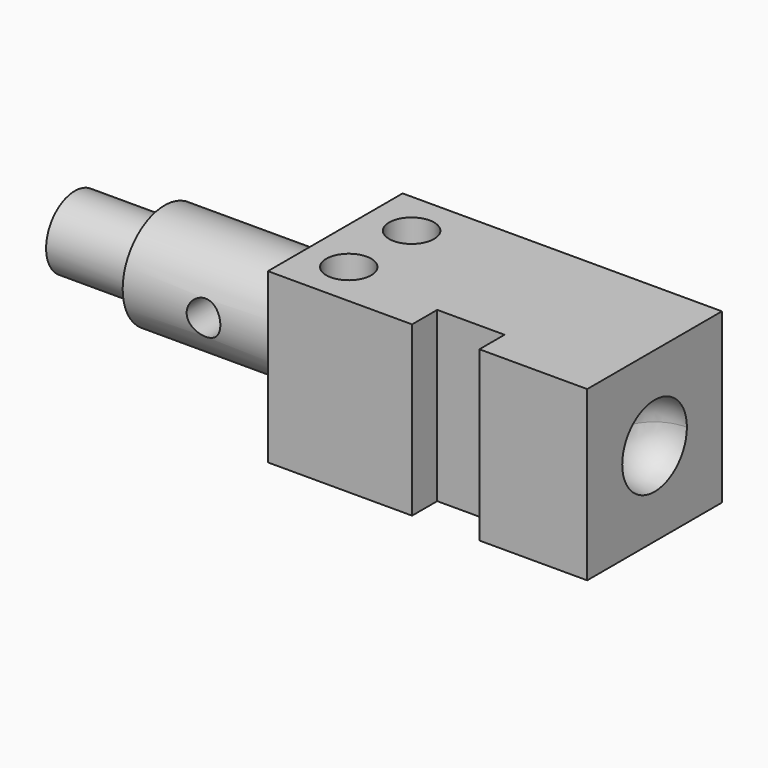
from build123d import *
from build123d import SkipClean  # not in build123d's __all__

# Parameters (mm, degrees)
F0_R      = 6.35
F1_DEPTH  = 47.625
F5_R      = 14.8376639977
F6_DEPTH  = 48.26
F7_R      = 10.16
F8_DEPTH  = 25.4
F10_R     = 4.7625
F11_DEPTH = 127
F9_R      = 2.286
F12_DEPTH = 44.083008926


with BuildPart() as f1:
    # F0 (on Top) → F1 (new body)
    with BuildSketch(Plane.XY):
        Polygon((0, 47.625), (0, 0), (40.767, 0), (40.767, 8.89), (59.817, 8.89), (59.817, 0), (90.297, 0), (90.297, 47.625), align=None)
        with Locations((12.7, 12.7)):
            Circle(F0_R, mode=Mode.SUBTRACT)
        with Locations((12.7, 34.925)):
            Circle(F0_R, mode=Mode.SUBTRACT)
    extrude(amount=F1_DEPTH)

    # F3 (on offset) → F4 (revolve, cut)
    with BuildSketch(Plane(origin=(0, 0, 23.8125), x_dir=(1, 0, 0), z_dir=(0, 0, -1))):
        with BuildLine():
            Line((90.297, -35.2425), (90.297, -12.3825))
            ThreePointArc((90.297, -12.3825), (78.867, -23.8125), (90.297, -35.2425))
        make_face()
    with SkipClean():  # cleaning this boolean's faces spoils the solid; the shape is the same uncleaned
        revolve(axis=Axis((90.297, 23.8125, 23.8125), (0, 1, 0)), mode=Mode.SUBTRACT)

    # F5 (on face) → F6 (join)
    with BuildSketch(Plane(origin=(0, 0, 0), x_dir=(0, -1, 0), z_dir=(-1, 0, 0))):
        with Locations((-23.8125, 23.8125)):
            Circle(F5_R)
    with SkipClean():  # cleaning this boolean's faces spoils the solid; the shape is the same uncleaned
        extrude(amount=F6_DEPTH)

    # F7 (on face) → F8 (join)
    with BuildSketch(Plane(origin=(-48.26, 0, 0), x_dir=(0, -1, 0), z_dir=(-1, 0, 0))):
        with Locations((-23.8125, 23.8125)):
            Circle(F7_R)
    with SkipClean():  # cleaning this boolean's faces spoils the solid; the shape is the same uncleaned
        extrude(amount=F8_DEPTH)

    # F10 (on Front) → F11 (cut)
    with BuildSketch(Plane.XZ):
        with Locations((-25.4, 23.8125)):
            Circle(F10_R)
    with SkipClean():  # cleaning this boolean's faces spoils the solid; the shape is the same uncleaned
        extrude(amount=-F11_DEPTH, mode=Mode.SUBTRACT)

    # F9 (on face) → F12 (cut, through all)
    with BuildSketch(Plane(origin=(-73.66, 0, 0), x_dir=(0, -1, 0), z_dir=(-1, 0, 0))):
        with Locations((-23.8125, 23.8125)):
            Circle(F9_R)
    with SkipClean():  # cleaning this boolean's faces spoils the solid; the shape is the same uncleaned
        extrude(amount=-F12_DEPTH, mode=Mode.SUBTRACT)


solid = f1.part
